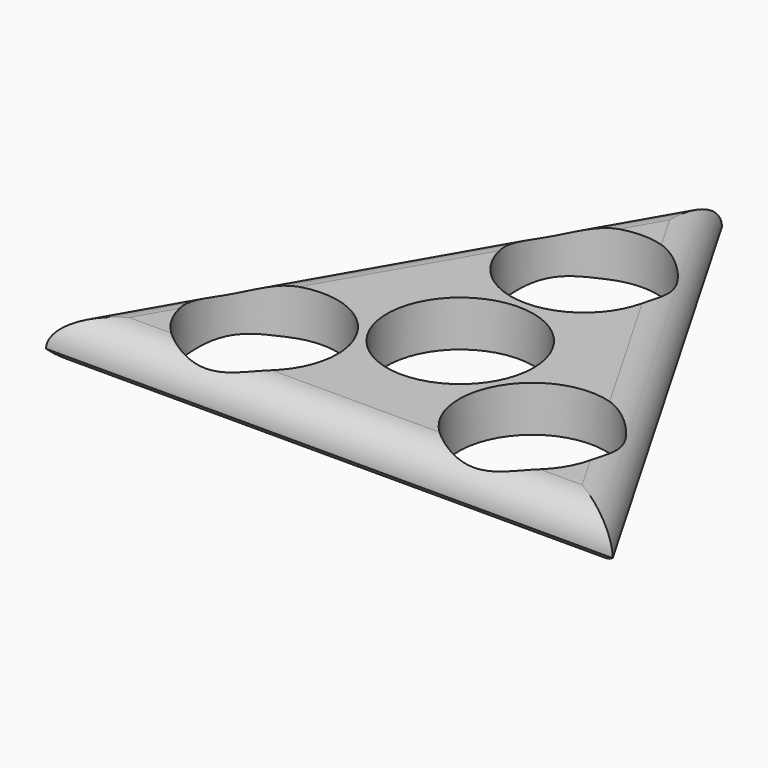
from build123d import *

# Parameters (mm, degrees)
F0_R        = 11.2
F1_DEPTH    = 7
F2_T1_DEPTH = 111.6025403784
F2_T3_DEPTH = 111.6025403784
F2_T5_DEPTH = 111.6025403784
F3_T1_DEPTH = 106.6025403784
F3_T3_DEPTH = 106.6025403784
F3_T5_DEPTH = 106.6025403784


# Not quite as in the source:
# - a fillet or chamfer that OpenCascade refuses, or shapes differently, is made with other operations: its cross-section is extruded or revolved along the edge and cut away or added


with BuildPart() as f1:
    # F0 (on Top) → F1 (new body)
    with BuildSketch(Plane.XY):
        Polygon((43.3012701892, -25), (0, 50), (-43.3012701892, -25), align=None)
        with Locations((-20.4962927973, -11.8335401639)):
            Circle(F0_R, mode=Mode.SUBTRACT)
        with Locations((20.4962927973, -11.8335401639)):
            Circle(F0_R, mode=Mode.SUBTRACT)
        Circle(F0_R, mode=Mode.SUBTRACT)
        with Locations((0, 23.6670803279)):
            Circle(F0_R, mode=Mode.SUBTRACT)
    extrude(amount=F1_DEPTH)

    # F2: fillet of radius 5 on 3 edges, made by hand

    # F2_s2 → F2_t1 (cut)
    with BuildSketch(Plane(origin=(27.9006350946, 48.3253175473, 0), x_dir=(0, 0, 1), z_dir=(-0.5, -0.8660254038, 0))):
        with BuildLine():
            ThreePointArc((2, 25), (5.5355339059, 23.5355339059), (7, 20))
            Line((7, 20), (7, 25))
            Line((7, 25), (2, 25))
        make_face()
    extrude(amount=F2_T1_DEPTH, mode=Mode.SUBTRACT)

    # F2_s4 → F2_t3 (cut)
    with BuildSketch(Plane.YZ.offset(-55.8012701892)):
        with BuildLine():
            ThreePointArc((-25, 2), (-23.5355339059, 5.5355339059), (-20, 7))
            Line((-20, 7), (-25, 7))
            Line((-25, 7), (-25, 2))
        make_face()
    extrude(amount=F2_T3_DEPTH, mode=Mode.SUBTRACT)

    # F2_s6 → F2_t5 (cut)
    with BuildSketch(Plane(origin=(27.9006350946, -48.3253175473, 0), x_dir=(0, 0, 1), z_dir=(-0.5, 0.8660254038, 0))):
        with BuildLine():
            ThreePointArc((2, 25), (5.5355339059, 23.5355339059), (7, 20))
            Line((7, 20), (7, 25))
            Line((7, 25), (2, 25))
        make_face()
    extrude(amount=F2_T5_DEPTH, mode=Mode.SUBTRACT)

    # F3: fillet of radius 5 on 3 edges, made by hand

    # F3_s2 → F3_t1 (cut)
    with BuildSketch(Plane(origin=(26.6506350946, -46.1602540378, 0), x_dir=(0, 0, 1), z_dir=(-0.5, 0.8660254038, 0))):
        with BuildLine():
            ThreePointArc((2, 25), (0.527864045, 23.2360679775), (0, 21))
            Line((0, 21), (0, 25))
            Line((0, 25), (2, 25))
        make_face()
    extrude(amount=F3_T1_DEPTH, mode=Mode.SUBTRACT)

    # F3_s4 → F3_t3 (cut)
    with BuildSketch(Plane.YZ.offset(-53.3012701892)):
        with BuildLine():
            ThreePointArc((-21, 0), (-23.2360679775, 0.527864045), (-25, 2))
            Line((-25, 2), (-25, 0))
            Line((-25, 0), (-21, 0))
        make_face()
    extrude(amount=F3_T3_DEPTH, mode=Mode.SUBTRACT)

    # F3_s6 → F3_t5 (cut)
    with BuildSketch(Plane(origin=(26.6506350946, 46.1602540378, 0), x_dir=(0, 0, 1), z_dir=(-0.5, -0.8660254038, 0))):
        with BuildLine():
            ThreePointArc((0, 21), (0.527864045, 23.2360679775), (2, 25))
            Line((2, 25), (0, 25))
            Line((0, 25), (0, 21))
        make_face()
    extrude(amount=F3_T5_DEPTH, mode=Mode.SUBTRACT)


solid = f1.part
